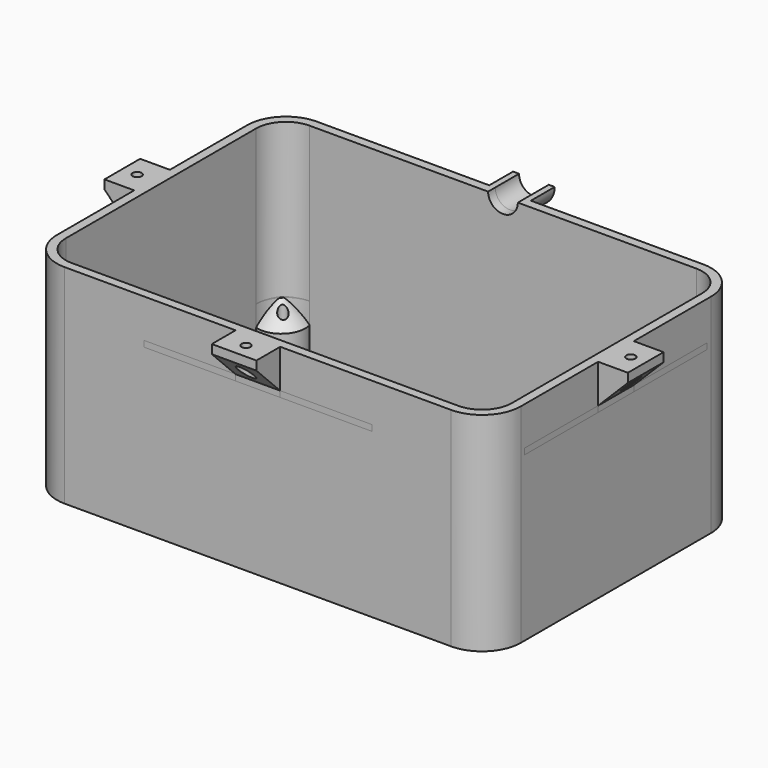
from build123d import *

# Parameters (mm, degrees)
F1_DEPTH        = 3
F2_DEPTH        = 70
F4_D            = 10
F4_DEPTH        = 5
F4_TIP          = 3.0043030951
F5_DEPTH        = 10
F6_W            = 10
F6_H            = 15
F6_W_2          = 15
F6_H_2          = 10
F7_DEPTH        = 15
F9_D            = 3
F9_DEPTH        = 15
F9_CBORE_D      = 5.5
F9_CBORE_DEPTH  = 12
F9_TIP          = 0.9012909285
F10_T4_DEPTH    = 76.7203917112
F10_T9_DEPTH    = 76.7203917112
F11_D           = 3
F11_DEPTH       = 5
F11_TIP         = 0.9012909285
F12_D           = 3
F12_DEPTH       = 5
F12_TIP         = 0.9012909285
F14_D           = 3
F14_DEPTH       = 15
F14_CBORE_D     = 5.5
F14_CBORE_DEPTH = 12
F14_TIP         = 0.9012909285
F15_T4_DEPTH    = 76.7203917112
F16_R           = 1.5
F17_DEPTH       = 15
F18_T4_ANGLE    = 359.64
F18_S5_R        = 10
F18_T6_DEPTH    = 64
F18_T10_ANGLE   = 359.64
F18_S11_R       = 10
F18_T12_DEPTH   = 64
F18_T16_ANGLE   = 359.64
F18_S17_R       = 10
F18_T18_DEPTH   = 64
F18_T22_ANGLE   = 359.64
F18_S23_R       = 10
F18_T24_DEPTH   = 64


# Not quite as in the source:
# - a fillet or chamfer that OpenCascade refuses, or shapes differently, is made with other operations: its cross-section is extruded or revolved along the edge and cut away or added


with BuildPart() as f1:
    # F0 (on Top) → F1 (new body)
    with BuildSketch(Plane.XY):
        with BuildLine():
            Line((83.5498416424, 80.5147014419), (-46.4501583576, 80.5147014419))
            ThreePointArc((-46.4501583576, 80.5147014419), (-53.5212261695, 77.5857692538), (-56.4501583576, 70.5147014419))
            Line((-56.4501583576, 70.5147014419), (-56.4501583576, -9.4852985581))
            ThreePointArc((-56.4501583576, -9.4852985581), (-53.5212261695, -16.5563663699), (-46.4501583576, -19.4852985581))
            Line((-46.4501583576, -19.4852985581), (83.5498416424, -19.4852985581))
            ThreePointArc((83.5498416424, -19.4852985581), (90.6209094542, -16.5563663699), (93.5498416424, -9.4852985581))
            Line((93.5498416424, -9.4852985581), (93.5498416424, 70.5147014419))
            ThreePointArc((93.5498416424, 70.5147014419), (90.6209094542, 77.5857692538), (83.5498416424, 80.5147014419))
        make_face()
        with BuildLine():
            ThreePointArc((-26.9749599767, 18.5104830032), (-22.4861700523, 16.5498687277), (-20.6405359507, 12.0125922225))
            Line((-20.6405359507, 12.0125922225), (-20.6405359507, 2.0125922225))
            ThreePointArc((-20.6405359507, 2.0125922225), (-22.4861700523, -2.5246842826), (-26.9749599767, -4.4852985581))
            ThreePointArc((-26.9749599767, -4.4852985581), (-31.6778124558, -2.6417736758), (-33.6405359507, 2.0125922225))
            Line((-33.6405359507, 2.0125922225), (-33.6405359507, 12.0125922225))
            ThreePointArc((-33.6405359507, 12.0125922225), (-31.6778124558, 16.6669581209), (-26.9749599767, 18.5104830032))
        make_face(mode=Mode.SUBTRACT)
        with BuildLine():
            Line((-15.1405359507, 2.0125922225), (-15.1405359507, 12.0125922225))
            ThreePointArc((-15.1405359507, 12.0125922225), (-13.1778124558, 16.6669581209), (-8.4749599767, 18.5104830032))
            ThreePointArc((-8.4749599767, 18.5104830032), (-3.9861700523, 16.5498687277), (-2.1405359507, 12.0125922225))
            Line((-2.1405359507, 12.0125922225), (-2.1405359507, 2.0125922225))
            ThreePointArc((-2.1405359507, 2.0125922225), (-3.9861700523, -2.5246842826), (-8.4749599767, -4.4852985581))
            ThreePointArc((-8.4749599767, -4.4852985581), (-13.1778124558, -2.6417736758), (-15.1405359507, 2.0125922225))
        make_face(mode=Mode.SUBTRACT)
        with BuildLine():
            ThreePointArc((16.3594640493, 2.0125922225), (14.5138299477, -2.5246842826), (10.0250400233, -4.4852985581))
            ThreePointArc((10.0250400233, -4.4852985581), (5.3221875442, -2.6417736758), (3.3594640493, 2.0125922225))
            Line((3.3594640493, 2.0125922225), (3.3594640493, 12.0125922225))
            ThreePointArc((3.3594640493, 12.0125922225), (5.3221875442, 16.6669581209), (10.0250400233, 18.5104830032))
            ThreePointArc((10.0250400233, 18.5104830032), (14.5138299477, 16.5498687277), (16.3594640493, 12.0125922225))
            Line((16.3594640493, 12.0125922225), (16.3594640493, 2.0125922225))
        make_face(mode=Mode.SUBTRACT)
        with BuildLine():
            ThreePointArc((34.8594640493, 2.0125922225), (33.0138299477, -2.5246842826), (28.5250400233, -4.4852985581))
            ThreePointArc((28.5250400233, -4.4852985581), (23.8221875442, -2.6417736758), (21.8594640493, 2.0125922225))
            Line((21.8594640493, 2.0125922225), (21.8594640493, 12.0125922225))
            ThreePointArc((21.8594640493, 12.0125922225), (23.8221875442, 16.6669581209), (28.5250400233, 18.5104830032))
            ThreePointArc((28.5250400233, 18.5104830032), (33.0138299477, 16.5498687277), (34.8594640493, 12.0125922225))
            Line((34.8594640493, 12.0125922225), (34.8594640493, 2.0125922225))
        make_face(mode=Mode.SUBTRACT)
        with BuildLine():
            ThreePointArc((53.3594640493, 2.0125922225), (51.5138299477, -2.5246842826), (47.0250400233, -4.4852985581))
            ThreePointArc((47.0250400233, -4.4852985581), (42.3221875442, -2.6417736758), (40.3594640493, 2.0125922225))
            Line((40.3594640493, 2.0125922225), (40.3594640493, 12.0125922225))
            ThreePointArc((40.3594640493, 12.0125922225), (42.3221875442, 16.6669581209), (47.0250400233, 18.5104830032))
            ThreePointArc((47.0250400233, 18.5104830032), (51.5138299477, 16.5498687277), (53.3594640493, 12.0125922225))
            Line((53.3594640493, 12.0125922225), (53.3594640493, 2.0125922225))
        make_face(mode=Mode.SUBTRACT)
        with BuildLine():
            ThreePointArc((71.8594640493, 2.0125922225), (70.0138299477, -2.5246842826), (65.5250400233, -4.4852985581))
            ThreePointArc((65.5250400233, -4.4852985581), (60.8221875442, -2.6417736758), (58.8594640493, 2.0125922225))
            Line((58.8594640493, 2.0125922225), (58.8594640493, 12.0125922225))
            ThreePointArc((58.8594640493, 12.0125922225), (60.8221875442, 16.6669581209), (65.5250400233, 18.5104830032))
            ThreePointArc((65.5250400233, 18.5104830032), (70.0138299477, 16.5498687277), (71.8594640493, 12.0125922225))
            Line((71.8594640493, 12.0125922225), (71.8594640493, 2.0125922225))
        make_face(mode=Mode.SUBTRACT)
    extrude(amount=F1_DEPTH)

    # F11
    with Locations(Plane(origin=(0, 0, 0), x_dir=(1, 0, 0), z_dir=(0, 0, -1))):
        with Locations((-33.6405359507, -28.5133267817), (73.8594640493, -18.5104830032)):
            Hole(F11_D / 2, depth=F11_DEPTH)
            with Locations((0, 0, -(F11_DEPTH + F11_TIP / 2))):  # 118° drill point
                Cone(0, F11_D / 2, F11_TIP, mode=Mode.SUBTRACT)

    # F12
    with Locations(Plane(origin=(0, 0, 0), x_dir=(1, 0, 0), z_dir=(0, 0, -1))):
        with Locations((88.5498416424, -75.5147014419), (-51.4501583576, -75.5147014419), (-51.4501583576, 14.4852985581), (88.5498416424, 14.4852985581)):
            Hole(F12_D / 2, depth=F12_DEPTH)
            with Locations((0, 0, -(F12_DEPTH + F12_TIP / 2))):  # 118° drill point
                Cone(0, F12_D / 2, F12_TIP, mode=Mode.SUBTRACT)


with BuildPart() as f2:
    # F0 (on Top) → F2 (new body)
    with BuildSketch(Plane.XY):
        with BuildLine():
            Line((-59.4501583576, 70.5147014419), (-59.4501583576, -9.4852985581))
            ThreePointArc((-59.4501583576, -9.4852985581), (-55.642546513, -18.6776867135), (-46.4501583576, -22.4852985581))
            Line((-46.4501583576, -22.4852985581), (83.5498416424, -22.4852985581))
            ThreePointArc((83.5498416424, -22.4852985581), (92.7422297978, -18.6776867135), (96.5498416424, -9.4852985581))
            Line((96.5498416424, -9.4852985581), (96.5498416424, 70.5147014419))
            ThreePointArc((96.5498416424, 70.5147014419), (92.7422297978, 79.7070895973), (83.5498416424, 83.5147014419))
            Line((83.5498416424, 83.5147014419), (-46.4501583576, 83.5147014419))
            ThreePointArc((-46.4501583576, 83.5147014419), (-55.642546513, 79.7070895973), (-59.4501583576, 70.5147014419))
        make_face()
        with BuildLine():
            ThreePointArc((-56.4501583576, 70.5147014419), (-53.5212261695, 77.5857692538), (-46.4501583576, 80.5147014419))
            Line((-46.4501583576, 80.5147014419), (83.5498416424, 80.5147014419))
            ThreePointArc((83.5498416424, 80.5147014419), (90.6209094542, 77.5857692538), (93.5498416424, 70.5147014419))
            Line((93.5498416424, 70.5147014419), (93.5498416424, -9.4852985581))
            ThreePointArc((93.5498416424, -9.4852985581), (90.6209094542, -16.5563663699), (83.5498416424, -19.4852985581))
            Line((83.5498416424, -19.4852985581), (-46.4501583576, -19.4852985581))
            ThreePointArc((-46.4501583576, -19.4852985581), (-53.5212261695, -16.5563663699), (-56.4501583576, -9.4852985581))
            Line((-56.4501583576, -9.4852985581), (-56.4501583576, 70.5147014419))
        make_face(mode=Mode.SUBTRACT)
    extrude(amount=F2_DEPTH)

    # F4
    with Locations(Plane(origin=(0, 83.5147014419, 0), x_dir=(-1, 0, 0), z_dir=(0, 1, 0))):
        with Locations((-18.5498416424, 70)):
            Hole(F4_D / 2, depth=F4_DEPTH)
            with Locations((0, 0, -(F4_DEPTH + F4_TIP / 2))):  # 118° drill point
                Cone(0, F4_D / 2, F4_TIP, mode=Mode.SUBTRACT)

    # F3 (on face) → F5 (join)
    with BuildSketch(Plane(origin=(0, 83.5147014419, 0), x_dir=(-1, 0, 0), z_dir=(0, 1, 0))):
        with BuildLine():
            Line((-11.5498416424, 70), (-13.5498416424, 70))
            ThreePointArc((-13.5498416424, 70), (-18.5498416424, 65), (-23.5498416424, 70))
            Line((-23.5498416424, 70), (-25.5498416424, 70))
            ThreePointArc((-25.5498416424, 70), (-18.5498416424, 63), (-11.5498416424, 70))
        make_face()
    extrude(amount=F5_DEPTH)

    # F6 (on face) → F7 (join)
    with BuildSketch(Plane.XY.offset(70)):
        with Locations((-64.4501583576, 30.5147014419)):
            Rectangle(F6_W, F6_H)
        with Locations((101.5498416424, 30.5147014419)):
            Rectangle(F6_W, F6_H)
        with Locations((18.5498416424, -27.4852985581)):
            Rectangle(F6_W_2, F6_H_2)
    extrude(amount=-F7_DEPTH)

    # F9
    with Locations(Plane(origin=(0, 0, 55), x_dir=(1, 0, 0), z_dir=(0, 0, -1))):
        with Locations((101.5498416424, -30.5147014419), (-64.4501583576, -30.5147014419)):
            CounterBoreHole(F9_D / 2, F9_CBORE_D / 2, F9_CBORE_DEPTH, depth=F9_DEPTH)
            with Locations((0, 0, -(F9_DEPTH + F9_TIP / 2))):  # 118° drill point
                Cone(0, F9_D / 2, F9_TIP, mode=Mode.SUBTRACT)

    # F10: chamfer of 12 on 2 edges, made by hand


with BuildPart() as f10_tool2:
    # F10_s3 → F10_t4 (new body)
    with BuildSketch(Plane.XZ.offset(-68.8748972975)):
        Polygon((-57.4501583576, 55), (-69.4501583576, 67), (-69.4501583576, 55), align=None)
    extrude(amount=F10_T4_DEPTH)

    split(bisect_by=Plane.YZ.offset(-59.4501583576), keep=Keep.BOTTOM)


with BuildPart() as f2_1:
    add(f2.part)

    # F10_t1: cut F10_tool2
    add(f10_tool2.part, mode=Mode.SUBTRACT)


with BuildPart() as f10_tool7:
    # F10_s8 → F10_t9 (new body)
    with BuildSketch(Plane.XZ.offset(7.8454944137)):
        Polygon((94.5498416424, 55), (106.5498416424, 67), (106.5498416424, 55), align=None)
    extrude(amount=-F10_T9_DEPTH)

    split(bisect_by=Plane.YZ.offset(96.5498416424), keep=Keep.TOP)


with BuildPart() as f2_2:
    add(f2_1.part)

    # F10_t6: cut F10_tool7
    add(f10_tool7.part, mode=Mode.SUBTRACT)

    # F14
    with Locations(Plane(origin=(0, 0, 55), x_dir=(1, 0, 0), z_dir=(0, 0, -1))):
        with Locations((18.5498416424, 27.4852985581)):
            CounterBoreHole(F14_D / 2, F14_CBORE_D / 2, F14_CBORE_DEPTH, depth=F14_DEPTH)
            with Locations((0, 0, -(F14_DEPTH + F14_TIP / 2))):  # 118° drill point
                Cone(0, F14_D / 2, F14_TIP, mode=Mode.SUBTRACT)

    # F15: chamfer of 12 on 1 edges, made by hand


with BuildPart() as f15_tool2:
    # F15_s3 → F15_t4 (new body)
    with BuildSketch(Plane.YZ.offset(-19.8103542132)):
        Polygon((-20.4852985581, 55), (-32.4852985581, 67), (-32.4852985581, 55), align=None)
    extrude(amount=F15_T4_DEPTH)

    split(bisect_by=Plane.XZ.offset(22.4852985581), keep=Keep.TOP)


with BuildPart() as f2_3:
    add(f2_2.part)

    # F15_t1: cut F15_tool2
    add(f15_tool2.part, mode=Mode.SUBTRACT)

    # F16 (on face) → F17 (join)
    with BuildSketch(Plane.XY.offset(3)):
        with BuildLine():
            ThreePointArc((-46.4501583576, 80.5147014419), (-53.5212261695, 77.5857692538), (-56.4501583576, 70.5147014419))
            ThreePointArc((-56.4501583576, 70.5147014419), (-48.493671068, 72.5582141523), (-46.4501583576, 80.5147014419))
        make_face()
        with Locations((-51.4501583576, 75.5147014419)):
            Circle(F16_R, mode=Mode.SUBTRACT)
        with BuildLine():
            ThreePointArc((93.5498416424, 70.5147014419), (90.6209094542, 77.5857692538), (83.5498416424, 80.5147014419))
            ThreePointArc((83.5498416424, 80.5147014419), (85.5933543528, 72.5582141523), (93.5498416424, 70.5147014419))
        make_face()
        with Locations((88.5498416424, 75.5147014419)):
            Circle(F16_R, mode=Mode.SUBTRACT)
        with BuildLine():
            ThreePointArc((93.5498416424, -9.4852985581), (85.5933543528, -11.5288112685), (83.5498416424, -19.4852985581))
            ThreePointArc((83.5498416424, -19.4852985581), (90.6209094542, -16.5563663699), (93.5498416424, -9.4852985581))
        make_face()
        with Locations((88.5498416424, -14.4852985581)):
            Circle(F16_R, mode=Mode.SUBTRACT)
        with BuildLine():
            ThreePointArc((-46.4501583576, -19.4852985581), (-48.493671068, -11.5288112685), (-56.4501583576, -9.4852985581))
            ThreePointArc((-56.4501583576, -9.4852985581), (-53.5212261695, -16.5563663699), (-46.4501583576, -19.4852985581))
        make_face()
        with Locations((-51.4501583576, -14.4852985581)):
            Circle(F16_R, mode=Mode.SUBTRACT)
    extrude(amount=F17_DEPTH)

    # F18: chamfer of 7 on 4 edges, made by hand


with BuildPart() as f18_tool2:
    # F18_s3 → F18_t4 (revolve)
    with BuildSketch(Plane(origin=(12.2017720091, 12.2786798698, 0), x_dir=(0, 0, 1), z_dir=(0.7048818539, 0.7093247296, 0))):
        with BuildLine():
            Line((10.8020101013, -101.8803459715), (18.1979898987, -94.484366174))
            Line((18.1979898987, -94.484366174), (18.3379898987, -94.484366174))
            ThreePointArc((18.3379898987, -94.484366174), (18.14, -98.0833611234), (18.14, -101.6823560728))
            Line((18.14, -101.6823560728), (18, -101.8223560728))
            ThreePointArc((18, -101.8223560728), (14.4010050506, -101.8223560728), (10.8020101013, -102.0203459715))
            Line((10.8020101013, -102.0203459715), (10.8020101013, -101.8803459715))
        make_face()
    revolve(axis=Axis((-54.199905154, 78.2644482383, 18), (0, 0, 1)), revolution_arc=F18_T4_ANGLE)

    # F18_s5 → F18_t6 (intersect, symmetric)
    with BuildSketch(Plane.XY.offset(16.2)):
        with Locations((-46.4501583576, 70.5147014419)):
            Circle(F18_S5_R)
    extrude(amount=F18_T6_DEPTH, both=True, mode=Mode.INTERSECT)


with BuildPart() as f2_4:
    add(f2_3.part)

    # F18_t1: cut F18_tool2
    add(f18_tool2.part, mode=Mode.SUBTRACT)


with BuildPart() as f18_tool8:
    # F18_s9 → F18_t10 (revolve)
    with BuildSketch(Plane(origin=(-18.6528729058, 18.5360401055, 0), x_dir=(0, 0, 1), z_dir=(-0.7093247296, 0.7048818539, 0))):
        with BuildLine():
            Line((10.8020101013, -58.697597047), (18.1979898987, -51.3016172495))
            Line((18.1979898987, -51.3016172495), (18.3379898987, -51.3016172495))
            ThreePointArc((18.3379898987, -51.3016172495), (18.14, -54.9006121989), (18.14, -58.4996071482))
            Line((18.14, -58.4996071482), (18, -58.6396071482))
            ThreePointArc((18, -58.6396071482), (14.4010050506, -58.6396071482), (10.8020101013, -58.837597047))
            Line((10.8020101013, -58.837597047), (10.8020101013, -58.697597047))
        make_face()
    revolve(axis=Axis((-54.199905154, -17.2350453545, 18), (0, 0, 1)), revolution_arc=F18_T10_ANGLE)

    # F18_s11 → F18_t12 (intersect, symmetric)
    with BuildSketch(Plane.XY.offset(16.2)):
        with Locations((-46.4501583576, -9.4852985581)):
            Circle(F18_S11_R)
    extrude(amount=F18_T12_DEPTH, both=True, mode=Mode.INTERSECT)


with BuildPart() as f2_5:
    add(f2_4.part)

    # F18_t7: cut F18_tool8
    add(f18_tool8.part, mode=Mode.SUBTRACT)


with BuildPart() as f18_tool14:
    # F18_s15 → F18_t16 (revolve)
    with BuildSketch(Plane(origin=(6.8051667659, -6.7625424102, 0), x_dir=(0, 0, 1), z_dir=(0.7093247296, -0.7048818539, 0))):
        with BuildLine():
            Line((10.8020101013, -128.138155278), (18.1979898987, -120.7421754805))
            Line((18.1979898987, -120.7421754805), (18.3379898987, -120.7421754805))
            ThreePointArc((18.3379898987, -120.7421754805), (18.14, -124.3411704299), (18.14, -127.9401653792))
            Line((18.14, -127.9401653792), (18, -128.0801653792))
            ThreePointArc((18, -128.0801653792), (14.4010050506, -128.0801653792), (10.8020101013, -128.278155278))
            Line((10.8020101013, -128.278155278), (10.8020101013, -128.138155278))
        make_face()
    revolve(axis=Axis((91.2995884388, 78.2644482383, 18), (0, 0, 1)), revolution_arc=F18_T16_ANGLE)

    # F18_s17 → F18_t18 (intersect, symmetric)
    with BuildSketch(Plane.XY.offset(16.2)):
        with Locations((83.5498416424, 70.5147014419)):
            Circle(F18_S17_R)
    extrude(amount=F18_T18_DEPTH, both=True, mode=Mode.INTERSECT)


with BuildPart() as f2_6:
    add(f2_5.part)

    # F18_t13: cut F18_tool14
    add(f18_tool14.part, mode=Mode.SUBTRACT)


with BuildPart() as f18_tool20:
    # F18_s21 → F18_t22 (revolve)
    with BuildSketch(Plane(origin=(36.7456174156, 36.9772253187, 0), x_dir=(0, 0, 1), z_dir=(-0.7048818539, -0.7093247296, 0))):
        with BuildLine():
            Line((10.8020101013, -85.1775501349), (18.1979898987, -77.7815703375))
            Line((18.1979898987, -77.7815703375), (18.3379898987, -77.7815703375))
            ThreePointArc((18.3379898987, -77.7815703375), (18.14, -81.3805652868), (18.14, -84.9795602362))
            Line((18.14, -84.9795602362), (18, -85.1195602362))
            ThreePointArc((18, -85.1195602362), (14.4010050506, -85.1195602362), (10.8020101013, -85.3175501349))
            Line((10.8020101013, -85.3175501349), (10.8020101013, -85.1775501349))
        make_face()
    revolve(axis=Axis((91.2995884388, -17.2350453545, 18), (0, 0, 1)), revolution_arc=F18_T22_ANGLE)

    # F18_s23 → F18_t24 (intersect, symmetric)
    with BuildSketch(Plane.XY.offset(16.2)):
        with Locations((83.5498416424, -9.4852985581)):
            Circle(F18_S23_R)
    extrude(amount=F18_T24_DEPTH, both=True, mode=Mode.INTERSECT)


with BuildPart() as f2_7:
    add(f2_6.part)

    # F18_t19: cut F18_tool20
    add(f18_tool20.part, mode=Mode.SUBTRACT)


solid = Compound([f1.part, f2_7.part])
